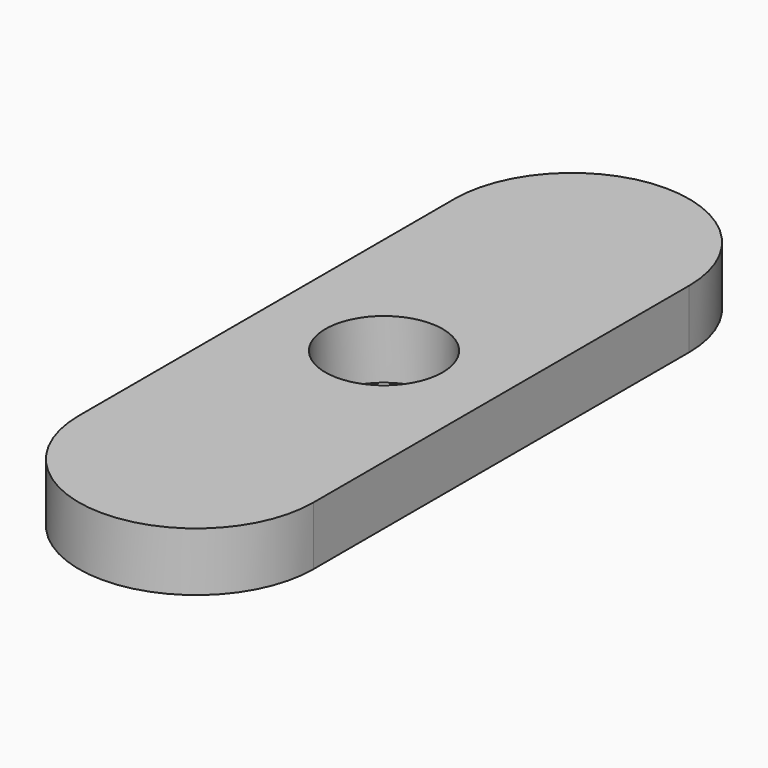
from build123d import *

# Parameters (mm, degrees)
F1_DEPTH = 1.25
F2_R     = 2.5
F3_DEPTH = 2.501


# Not quite as in the source:
# - a feature names something its author has since deleted; it is built from what else it names


with BuildPart() as f1:
    # F0 (on Top) → F1 (new body, symmetric)
    with BuildSketch(Plane.XY):
        with BuildLine():
            Line((-5, 10), (-5, 0))
            Line((-5, 0), (5, 0))
            Line((5, 0), (5, 10))
            ThreePointArc((5, 10), (0, 5), (-5, 10))
        make_face()
        with BuildLine():
            Line((5, 0), (-5, 0))
            Line((-5, 0), (-5, -10))
            ThreePointArc((-5, -10), (0, -5), (5, -10))
            Line((5, -10), (5, 0))
        make_face()
        with BuildLine():
            ThreePointArc((5, 10), (0, 15), (-5, 10))
            ThreePointArc((-5, 10), (0, 5), (5, 10))
        make_face()
        with BuildLine():
            ThreePointArc((5, -10), (0, -5), (-5, -10))
            ThreePointArc((-5, -10), (0, -15), (5, -10))
        make_face()
    extrude(amount=F1_DEPTH, both=True)

    # F2 (on face) → F3 (cut, through all)
    with BuildSketch(Plane.XY.offset(1.25)):
        Circle(F2_R)
    extrude(amount=-F3_DEPTH, mode=Mode.SUBTRACT)


solid = f1.part
